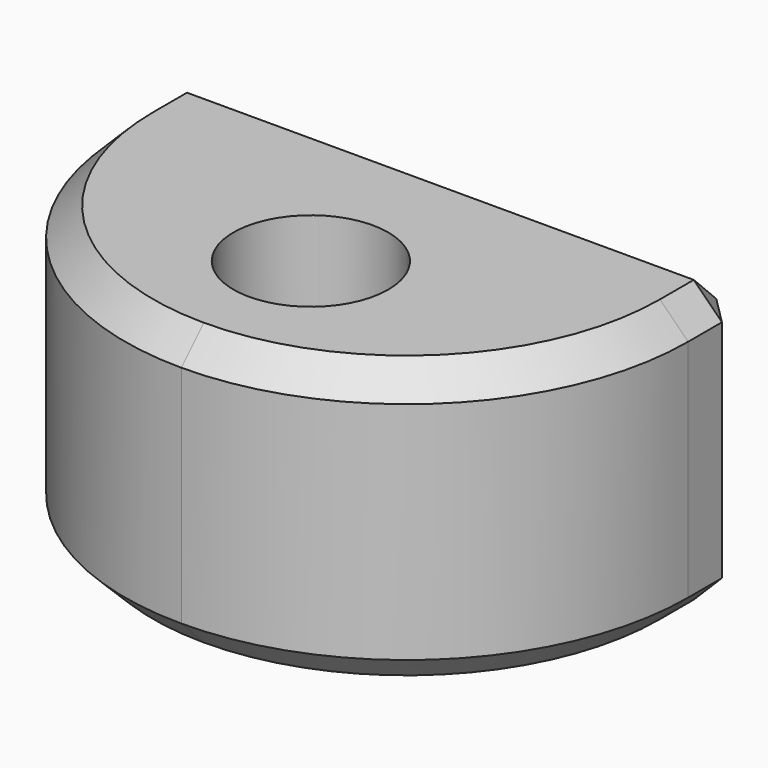
from build123d import *

# Parameters (mm, degrees)
F0_W     = 20
F0_H     = 10
F1_DEPTH = 12.5
F2_R     = 2.75
F3_DEPTH = 10
F4_R     = 9.99999
F5_SIZE  = 1


# Not quite as in the source:
# - a fillet or chamfer is up to 0.001 mm smaller than in the source, because OpenCascade refuses the exact size


with BuildPart() as f1:
    # F0 (on Front) → F1 (new body)
    with BuildSketch(Plane.XZ):
        with Locations((10, 5)):
            Rectangle(F0_W, F0_H)
    extrude(amount=F1_DEPTH)

    # F2 (on face) → F3 (cut, through all)
    with BuildSketch(Plane.XY.offset(10)):
        with Locations((10, -6.75)):
            Circle(F2_R)
    extrude(amount=-F3_DEPTH, mode=Mode.SUBTRACT)

    # F4 (radius 10 in the source; OpenCascade refuses exactly that, so slightly less here)
    f4_edges = [f1.edges().sort_by_distance(p)[0] for p in [
        (0, -12.5, 5),
        (20, -12.5, 5),
    ]]
    fillet(f4_edges, radius=F4_R)

    # F5
    f5_edges = [f1.edges().sort_by_distance(p)[0] for p in [
        (17.071071, -9.571071, 0),
        (10.00001, -12.5, 5),
        (20, -2.50001, 5),
        (17.071071, -9.571071, 10),
        (0, 0, 5),
        (10, 0, 0),
        (20, 0, 5),
        (10, 0, 10),
    ]]
    chamfer(f5_edges, length=F5_SIZE)


solid = f1.part
